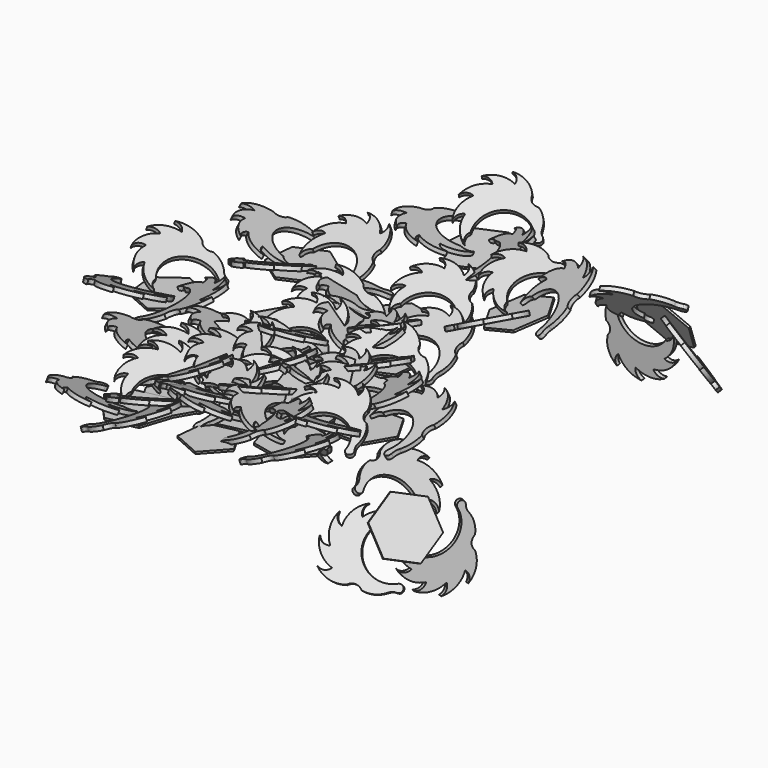
from build123d import *

# Parameters (mm, degrees)
F2_DEPTH  = 1
F3_DEPTH  = 1
F5_COUNT  = 5
F5_ANGLE  = 288
F8_DEPTH  = 2
F9_R      = 5
F11_ANGLE = 65
F12_COUNT = 5
F12_ANGLE = 288
F14_COUNT = 3
F14_ANGLE = 240
F15_COUNT = 5
F15_ANGLE = 288
F16_COUNT = 2
F16_ANGLE = 120
F17_COUNT = 3
F17_ANGLE = 240
F21_COUNT = 3
F21_ANGLE = 144
F25_COUNT = 3
F25_ANGLE = 144
F28_COUNT = 2
F28_ANGLE = 120
F31_COUNT = 3
F31_ANGLE = 144
F35_COUNT = 3
F35_ANGLE = 240
F39_COUNT = 3
F39_ANGLE = 144
F43_COUNT = 3
F43_ANGLE = 144
F47_COUNT = 2
F47_ANGLE = 120
F51_COUNT = 2
F51_ANGLE = 120
F55_COUNT = 2
F55_ANGLE = 120
F59_COUNT = 2
F59_ANGLE = 120


with BuildPart() as f2:
    # F0 (on Top) → F2 (new body)
    with BuildSketch(Plane.XY):
        Polygon((0, -10.3228644035), (7.5, -10.3228644035), (12.1352549156, 3.9429833409), (0, 12.7597621253), align=None)
        Polygon((-7.5, -10.3228644035), (0, -10.3228644035), (0, 12.7597621253), (-12.1352549156, 3.9429833409), align=None)
    extrude(amount=-F2_DEPTH)


with BuildPart() as f3:
    # F1 (on Top) → F3 (new body)
    with BuildSketch(Plane.XY):
        Polygon((32.2091731064, -18.3513614234), (36.844428022, -4.085513679), (26.8074689266, 7.0616587032), (12.1352549156, 3.9429833409), (7.5, -10.3228644035), (17.5369590954, -21.4700367857), align=None)
    extrude(amount=-F3_DEPTH)


with BuildPart() as f5_1:
    # F5: instance of F3
    add(f3.part.rotate(Axis((0, 0, 3.8664315362), (0, 0, 1)), 1 * F5_ANGLE / (F5_COUNT - 1)))


with BuildPart() as f5_2:
    # F5: instance of F3
    add(f3.part.rotate(Axis((0, 0, 3.8664315362), (0, 0, 1)), 2 * F5_ANGLE / (F5_COUNT - 1)))


with BuildPart() as f5_3:
    # F5: instance of F3
    add(f3.part.rotate(Axis((0, 0, 3.8664315362), (0, 0, 1)), 3 * F5_ANGLE / (F5_COUNT - 1)))


with BuildPart() as f5_4:
    # F5: instance of F3
    add(f3.part.rotate(Axis((0, 0, 3.8664315362), (0, 0, 1)), 4 * F5_ANGLE / (F5_COUNT - 1)))


with BuildPart() as f8:
    # F7 (on Right) → F8 (new body)
    with BuildSketch(Plane.YZ):
        with BuildLine():
            ThreePointArc((-24.95999832, 7.9226027528), (-9.4652729948, 14.9790762842), (-1.371596125, 0))
            ThreePointArc((-1.371596125, 0), (1.2710572909, -2.1110060804), (1.0658705895, 1.265065922))
            ThreePointArc((1.0658705895, 1.265065922), (3.462744203, 7.3677169674), (2.5001799222, 13.8531485572))
            ThreePointArc((2.5001799222, 13.8531485572), (0.2653261107, 16.5218708667), (0.7903517664, 19.9629460452))
            ThreePointArc((0.7903517664, 19.9629460452), (-0.5397085451, 26.9271758786), (-5.3926714222, 32.0961514944))
            ThreePointArc((-5.3926714222, 32.0961514944), (-4.1335314331, 29.2501097622), (-5.1634487101, 26.3133330502))
            ThreePointArc((-5.1634487101, 26.3133330502), (-10.3329616952, 31.1657235024), (-17.2973387723, 32.49501261))
            ThreePointArc((-17.2973387723, 32.49501261), (-14.6058117652, 30.9326203981), (-13.7128383045, 27.9513479429))
            ThreePointArc((-13.7128383045, 27.9513479429), (-20.7472257083, 28.8384507879), (-27.1628616524, 25.8203101291))
            ThreePointArc((-27.1628616524, 25.8203101291), (-24.0670194624, 26.1383481587), (-21.5922407749, 24.2513247085))
            ThreePointArc((-21.5922407749, 24.2513247085), (-27.8046056991, 20.834296811), (-31.220945639, 14.6215535346))
            ThreePointArc((-31.220945639, 14.6215535346), (-28.9032947589, 16.6985420881), (-25.7919921886, 16.6265464632))
            ThreePointArc((-25.7919921886, 16.6265464632), (-28.8094223827, 10.2105763396), (-27.9215405786, 3.1762872138))
            ThreePointArc((-27.9215405786, 3.1762872138), (-27.3380736099, 6.1093327886), (-24.95999832, 7.9226027528))
        make_face()
    extrude(amount=-F8_DEPTH)

    # F9
    f9_edges = [f8.edges().sort_by_distance(p)[0] for p in [
        (-1, 1.065871, 1.265066),
    ]]
    fillet(f9_edges, radius=F9_R)


with BuildPart() as f8_1:
    # F11: moved
    add(f8.part.rotate(Axis((0, -11.6566227302, 0), (0, -1, 0)), F11_ANGLE))


with BuildPart() as f12_1:
    # F12: instance of F8
    add(f8_1.part.rotate(Axis((0, 0, 14.2103461549), (0, 0, 1)), 1 * F12_ANGLE / (F12_COUNT - 1)))


with BuildPart() as f12_2:
    # F12: instance of F8
    add(f8_1.part.rotate(Axis((0, 0, 14.2103461549), (0, 0, 1)), 2 * F12_ANGLE / (F12_COUNT - 1)))


with BuildPart() as f12_3:
    # F12: instance of F8
    add(f8_1.part.rotate(Axis((0, 0, 14.2103461549), (0, 0, 1)), 3 * F12_ANGLE / (F12_COUNT - 1)))


with BuildPart() as f12_4:
    # F12: instance of F8
    add(f8_1.part.rotate(Axis((0, 0, 14.2103461549), (0, 0, 1)), 4 * F12_ANGLE / (F12_COUNT - 1)))


with BuildPart() as f14_1:
    # F14: instance of F8
    add(f8_1.part.rotate(Axis((0, -23.3132454603, 7.7419117889), (0, 0, 1)), 1 * F14_ANGLE / (F14_COUNT - 1)))


with BuildPart() as f14_2:
    # F14: instance of F8
    add(f8_1.part.rotate(Axis((0, -23.3132454603, 7.7419117889), (0, 0, 1)), 2 * F14_ANGLE / (F14_COUNT - 1)))


with BuildPart() as f15_1:
    # F15: instance of F14_2
    add(f14_2.part.rotate(Axis((0, 0, 14.2103461549), (0, 0, 1)), 1 * F15_ANGLE / (F15_COUNT - 1)))


with BuildPart() as f15_2:
    # F15: instance of F14_2
    add(f14_2.part.rotate(Axis((0, 0, 14.2103461549), (0, 0, 1)), 2 * F15_ANGLE / (F15_COUNT - 1)))


with BuildPart() as f15_3:
    # F15: instance of F14_2
    add(f14_2.part.rotate(Axis((0, 0, 14.2103461549), (0, 0, 1)), 3 * F15_ANGLE / (F15_COUNT - 1)))


with BuildPart() as f15_4:
    # F15: instance of F14_2
    add(f14_2.part.rotate(Axis((0, 0, 14.2103461549), (0, 0, 1)), 4 * F15_ANGLE / (F15_COUNT - 1)))


with BuildPart() as f15_5:
    # F15: instance of F14_1
    add(f14_1.part.rotate(Axis((0, 0, 14.2103461549), (0, 0, 1)), 1 * F15_ANGLE / (F15_COUNT - 1)))


with BuildPart() as f15_6:
    # F15: instance of F14_1
    add(f14_1.part.rotate(Axis((0, 0, 14.2103461549), (0, 0, 1)), 2 * F15_ANGLE / (F15_COUNT - 1)))


with BuildPart() as f15_7:
    # F15: instance of F14_1
    add(f14_1.part.rotate(Axis((0, 0, 14.2103461549), (0, 0, 1)), 3 * F15_ANGLE / (F15_COUNT - 1)))


with BuildPart() as f15_8:
    # F15: instance of F14_1
    add(f14_1.part.rotate(Axis((0, 0, 14.2103461549), (0, 0, 1)), 4 * F15_ANGLE / (F15_COUNT - 1)))


with BuildPart() as f16_1:
    # F16: instance of F3
    add(f3.part.rotate(Axis((0, -23.3132454603, 7.7419117889), (0, 0, -1)), 1 * F16_ANGLE / (F16_COUNT - 1)))


with BuildPart() as f16_2:
    # F16: instance of F15_5
    add(f15_5.part.rotate(Axis((0, -23.3132454603, 7.7419117889), (0, 0, -1)), 1 * F16_ANGLE / (F16_COUNT - 1)))


with BuildPart() as f16_3:
    # F16: instance of F12_1
    add(f12_1.part.rotate(Axis((0, -23.3132454603, 7.7419117889), (0, 0, -1)), 1 * F16_ANGLE / (F16_COUNT - 1)))


with BuildPart() as f16_4:
    # F16: instance of F15_1
    add(f15_1.part.rotate(Axis((0, -23.3132454603, 7.7419117889), (0, 0, -1)), 1 * F16_ANGLE / (F16_COUNT - 1)))


with BuildPart() as f17_1:
    # F17: instance of F2
    add(f2.part.rotate(Axis((0, -23.3132454603, 7.7419117889), (0, 0, 1)), 1 * F17_ANGLE / (F17_COUNT - 1)))


with BuildPart() as f17_2:
    # F17: instance of F2
    add(f2.part.rotate(Axis((0, -23.3132454603, 7.7419117889), (0, 0, 1)), 2 * F17_ANGLE / (F17_COUNT - 1)))


with BuildPart() as f17_3:
    # F17: instance of F12_2
    add(f12_2.part.rotate(Axis((0, -23.3132454603, 7.7419117889), (0, 0, 1)), 1 * F17_ANGLE / (F17_COUNT - 1)))


with BuildPart() as f17_4:
    # F17: instance of F12_2
    add(f12_2.part.rotate(Axis((0, -23.3132454603, 7.7419117889), (0, 0, 1)), 2 * F17_ANGLE / (F17_COUNT - 1)))


with BuildPart() as f17_5:
    # F17: instance of F12_3
    add(f12_3.part.rotate(Axis((0, -23.3132454603, 7.7419117889), (0, 0, 1)), 1 * F17_ANGLE / (F17_COUNT - 1)))


with BuildPart() as f17_6:
    # F17: instance of F12_3
    add(f12_3.part.rotate(Axis((0, -23.3132454603, 7.7419117889), (0, 0, 1)), 2 * F17_ANGLE / (F17_COUNT - 1)))


with BuildPart() as f21_1:
    # F21: instance of F16_1
    add(f16_1.part.rotate(Axis((-17.4362215627, -33.3800526732, 1.1737770455), (0, 0, -1)), 1 * F21_ANGLE / (F21_COUNT - 1)))


with BuildPart() as f21_2:
    # F21: instance of F16_1
    add(f16_1.part.rotate(Axis((-17.4362215627, -33.3800526732, 1.1737770455), (0, 0, -1)), 2 * F21_ANGLE / (F21_COUNT - 1)))


with BuildPart() as f21_3:
    # F21: instance of F16_3
    add(f16_3.part.rotate(Axis((-17.4362215627, -33.3800526732, 1.1737770455), (0, 0, -1)), 1 * F21_ANGLE / (F21_COUNT - 1)))


with BuildPart() as f21_4:
    # F21: instance of F16_3
    add(f16_3.part.rotate(Axis((-17.4362215627, -33.3800526732, 1.1737770455), (0, 0, -1)), 2 * F21_ANGLE / (F21_COUNT - 1)))


with BuildPart() as f21_5:
    # F21: instance of F16_4
    add(f16_4.part.rotate(Axis((-17.4362215627, -33.3800526732, 1.1737770455), (0, 0, -1)), 1 * F21_ANGLE / (F21_COUNT - 1)))


with BuildPart() as f21_6:
    # F21: instance of F16_4
    add(f16_4.part.rotate(Axis((-17.4362215627, -33.3800526732, 1.1737770455), (0, 0, -1)), 2 * F21_ANGLE / (F21_COUNT - 1)))


with BuildPart() as f21_7:
    # F21: instance of F16_2
    add(f16_2.part.rotate(Axis((-17.4362215627, -33.3800526732, 1.1737770455), (0, 0, -1)), 1 * F21_ANGLE / (F21_COUNT - 1)))


with BuildPart() as f21_8:
    # F21: instance of F16_2
    add(f16_2.part.rotate(Axis((-17.4362215627, -33.3800526732, 1.1737770455), (0, 0, -1)), 2 * F21_ANGLE / (F21_COUNT - 1)))


with BuildPart() as f25_1:
    # F25: instance of F3
    add(f3.part.rotate(Axis((17.4362215627, -33.3800526732, 3.6553055273), (0, 0, -1)), 1 * F25_ANGLE / (F25_COUNT - 1)))


with BuildPart() as f25_2:
    # F25: instance of F3
    add(f3.part.rotate(Axis((17.4362215627, -33.3800526732, 3.6553055273), (0, 0, -1)), 2 * F25_ANGLE / (F25_COUNT - 1)))


with BuildPart() as f25_3:
    # F25: instance of F15_1
    add(f15_1.part.rotate(Axis((17.4362215627, -33.3800526732, 3.6553055273), (0, 0, -1)), 1 * F25_ANGLE / (F25_COUNT - 1)))


with BuildPart() as f25_4:
    # F25: instance of F15_1
    add(f15_1.part.rotate(Axis((17.4362215627, -33.3800526732, 3.6553055273), (0, 0, -1)), 2 * F25_ANGLE / (F25_COUNT - 1)))


with BuildPart() as f25_5:
    # F25: instance of F12_1
    add(f12_1.part.rotate(Axis((17.4362215627, -33.3800526732, 3.6553055273), (0, 0, -1)), 1 * F25_ANGLE / (F25_COUNT - 1)))


with BuildPart() as f25_6:
    # F25: instance of F12_1
    add(f12_1.part.rotate(Axis((17.4362215627, -33.3800526732, 3.6553055273), (0, 0, -1)), 2 * F25_ANGLE / (F25_COUNT - 1)))


with BuildPart() as f25_7:
    # F25: instance of F15_5
    add(f15_5.part.rotate(Axis((17.4362215627, -33.3800526732, 3.6553055273), (0, 0, -1)), 1 * F25_ANGLE / (F25_COUNT - 1)))


with BuildPart() as f25_8:
    # F25: instance of F15_5
    add(f15_5.part.rotate(Axis((17.4362215627, -33.3800526732, 3.6553055273), (0, 0, -1)), 2 * F25_ANGLE / (F25_COUNT - 1)))


with BuildPart() as f28_1:
    # F28: instance of F17_2
    add(f17_2.part.rotate(Axis((0, -50.5694742615, 7.2258593382), (0, 0, -1)), 1 * F28_ANGLE / (F28_COUNT - 1)))


with BuildPart() as f31_1:
    # F31: instance of F25_2
    add(f25_2.part.rotate(Axis((0, -75.8542113922, -11.0916886207), (0, 0, 1)), 1 * F31_ANGLE / (F31_COUNT - 1)))


with BuildPart() as f31_2:
    # F31: instance of F25_2
    add(f25_2.part.rotate(Axis((0, -75.8542113922, -11.0916886207), (0, 0, 1)), 2 * F31_ANGLE / (F31_COUNT - 1)))


with BuildPart() as f31_3:
    # F31: instance of F25_4
    add(f25_4.part.rotate(Axis((0, -75.8542113922, -11.0916886207), (0, 0, 1)), 1 * F31_ANGLE / (F31_COUNT - 1)))


with BuildPart() as f31_4:
    # F31: instance of F25_4
    add(f25_4.part.rotate(Axis((0, -75.8542113922, -11.0916886207), (0, 0, 1)), 2 * F31_ANGLE / (F31_COUNT - 1)))


with BuildPart() as f31_5:
    # F31: instance of F25_6
    add(f25_6.part.rotate(Axis((0, -75.8542113922, -11.0916886207), (0, 0, 1)), 1 * F31_ANGLE / (F31_COUNT - 1)))


with BuildPart() as f31_6:
    # F31: instance of F25_6
    add(f25_6.part.rotate(Axis((0, -75.8542113922, -11.0916886207), (0, 0, 1)), 2 * F31_ANGLE / (F31_COUNT - 1)))


with BuildPart() as f31_7:
    # F31: instance of F17_4
    add(f17_4.part.rotate(Axis((0, -75.8542113922, -11.0916886207), (0, 0, 1)), 1 * F31_ANGLE / (F31_COUNT - 1)))


with BuildPart() as f31_8:
    # F31: instance of F17_4
    add(f17_4.part.rotate(Axis((0, -75.8542113922, -11.0916886207), (0, 0, 1)), 2 * F31_ANGLE / (F31_COUNT - 1)))


with BuildPart() as f35_1:
    # F35: instance of F2
    add(f2.part.rotate(Axis((-13.7031818646, 18.8608117714, 14.763216387), (0, 0, -1)), 1 * F35_ANGLE / (F35_COUNT - 1)))


with BuildPart() as f35_2:
    # F35: instance of F2
    add(f2.part.rotate(Axis((-13.7031818646, 18.8608117714, 14.763216387), (0, 0, -1)), 2 * F35_ANGLE / (F35_COUNT - 1)))


with BuildPart() as f39_1:
    # F39: instance of F21_2
    add(f21_2.part.rotate(Axis((-36.888714927, 16.4239140497, 16.806895229), (0, 0, -1)), 1 * F39_ANGLE / (F39_COUNT - 1)))


with BuildPart() as f39_2:
    # F39: instance of F21_2
    add(f21_2.part.rotate(Axis((-36.888714927, 16.4239140497, 16.806895229), (0, 0, -1)), 2 * F39_ANGLE / (F39_COUNT - 1)))


with BuildPart() as f39_3:
    # F39: instance of F21_6
    add(f21_6.part.rotate(Axis((-36.888714927, 16.4239140497, 16.806895229), (0, 0, -1)), 1 * F39_ANGLE / (F39_COUNT - 1)))


with BuildPart() as f39_4:
    # F39: instance of F21_6
    add(f21_6.part.rotate(Axis((-36.888714927, 16.4239140497, 16.806895229), (0, 0, -1)), 2 * F39_ANGLE / (F39_COUNT - 1)))


with BuildPart() as f39_5:
    # F39: instance of F21_4
    add(f21_4.part.rotate(Axis((-36.888714927, 16.4239140497, 16.806895229), (0, 0, -1)), 1 * F39_ANGLE / (F39_COUNT - 1)))


with BuildPart() as f39_6:
    # F39: instance of F21_4
    add(f21_4.part.rotate(Axis((-36.888714927, 16.4239140497, 16.806895229), (0, 0, -1)), 2 * F39_ANGLE / (F39_COUNT - 1)))


with BuildPart() as f39_7:
    # F39: instance of F17_3
    add(f17_3.part.rotate(Axis((-36.888714927, 16.4239140497, 16.806895229), (0, 0, -1)), 1 * F39_ANGLE / (F39_COUNT - 1)))


with BuildPart() as f39_8:
    # F39: instance of F17_3
    add(f17_3.part.rotate(Axis((-36.888714927, 16.4239140497, 16.806895229), (0, 0, -1)), 2 * F39_ANGLE / (F39_COUNT - 1)))


with BuildPart() as f43_1:
    # F43: instance of F39_2
    add(f39_2.part.rotate(Axis((-8.0111221618, 39.3528699367, 26.0918540489), (0.1436912512, 0.0305425183, -0.9891511406)), 1 * F43_ANGLE / (F43_COUNT - 1)))


with BuildPart() as f43_2:
    # F43: instance of F39_2
    add(f39_2.part.rotate(Axis((-8.0111221618, 39.3528699367, 26.0918540489), (0.1436912512, 0.0305425183, -0.9891511406)), 2 * F43_ANGLE / (F43_COUNT - 1)))


with BuildPart() as f43_3:
    # F43: instance of F39_6
    add(f39_6.part.rotate(Axis((-8.0111221618, 39.3528699367, 26.0918540489), (0.1436912512, 0.0305425183, -0.9891511406)), 1 * F43_ANGLE / (F43_COUNT - 1)))


with BuildPart() as f43_4:
    # F43: instance of F39_6
    add(f39_6.part.rotate(Axis((-8.0111221618, 39.3528699367, 26.0918540489), (0.1436912512, 0.0305425183, -0.9891511406)), 2 * F43_ANGLE / (F43_COUNT - 1)))


with BuildPart() as f43_5:
    # F43: instance of F39_8
    add(f39_8.part.rotate(Axis((-8.0111221618, 39.3528699367, 26.0918540489), (0.1436912512, 0.0305425183, -0.9891511406)), 1 * F43_ANGLE / (F43_COUNT - 1)))


with BuildPart() as f43_6:
    # F43: instance of F39_8
    add(f39_8.part.rotate(Axis((-8.0111221618, 39.3528699367, 26.0918540489), (0.1436912512, 0.0305425183, -0.9891511406)), 2 * F43_ANGLE / (F43_COUNT - 1)))


with BuildPart() as f43_7:
    # F43: instance of F39_4
    add(f39_4.part.rotate(Axis((-8.0111221618, 39.3528699367, 26.0918540489), (0.1436912512, 0.0305425183, -0.9891511406)), 1 * F43_ANGLE / (F43_COUNT - 1)))


with BuildPart() as f43_8:
    # F43: instance of F39_4
    add(f39_4.part.rotate(Axis((-8.0111221618, 39.3528699367, 26.0918540489), (0.1436912512, 0.0305425183, -0.9891511406)), 2 * F43_ANGLE / (F43_COUNT - 1)))


with BuildPart() as f47_1:
    # F47: instance of F21_2
    add(f21_2.part.rotate(Axis((-92.9675551418, 6.3909135689, 0), (0.9981475566, 0.0608395868, 0)), 1 * F47_ANGLE / (F47_COUNT - 1)))


with BuildPart() as f47_2:
    # F47: instance of F21_4
    add(f21_4.part.rotate(Axis((-92.9675551418, 6.3909135689, 0), (0.9981475566, 0.0608395868, 0)), 1 * F47_ANGLE / (F47_COUNT - 1)))


with BuildPart() as f47_3:
    # F47: instance of F21_6
    add(f21_6.part.rotate(Axis((-92.9675551418, 6.3909135689, 0), (0.9981475566, 0.0608395868, 0)), 1 * F47_ANGLE / (F47_COUNT - 1)))


with BuildPart() as f47_4:
    # F47: instance of F17_3
    add(f17_3.part.rotate(Axis((-92.9675551418, 6.3909135689, 0), (0.9981475566, 0.0608395868, 0)), 1 * F47_ANGLE / (F47_COUNT - 1)))


with BuildPart() as f51_1:
    # F51: instance of F15_5
    add(f15_5.part.rotate(Axis((54.8325005267, -26.1451923699, 0), (-0.5517624006, -0.8340013509, 0)), 1 * F51_ANGLE / (F51_COUNT - 1)))


with BuildPart() as f51_2:
    # F51: instance of F12_1
    add(f12_1.part.rotate(Axis((54.8325005267, -26.1451923699, 0), (-0.5517624006, -0.8340013509, 0)), 1 * F51_ANGLE / (F51_COUNT - 1)))


with BuildPart() as f51_3:
    # F51: instance of F15_1
    add(f15_1.part.rotate(Axis((54.8325005267, -26.1451923699, 0), (-0.5517624006, -0.8340013509, 0)), 1 * F51_ANGLE / (F51_COUNT - 1)))


with BuildPart() as f51_4:
    # F51: instance of F3
    add(f3.part.rotate(Axis((54.8325005267, -26.1451923699, 0), (-0.5517624006, -0.8340013509, 0)), 1 * F51_ANGLE / (F51_COUNT - 1)))


with BuildPart() as f55_1:
    # F55: instance of F25_2
    add(f25_2.part.rotate(Axis((-16.1490089096, -14.5711711071, -22.7108248674), (0, 0, 1)), 1 * F55_ANGLE / (F55_COUNT - 1)))


with BuildPart() as f55_2:
    # F55: instance of F25_4
    add(f25_4.part.rotate(Axis((-16.1490089096, -14.5711711071, -22.7108248674), (0, 0, 1)), 1 * F55_ANGLE / (F55_COUNT - 1)))


with BuildPart() as f55_3:
    # F55: instance of F25_6
    add(f25_6.part.rotate(Axis((-16.1490089096, -14.5711711071, -22.7108248674), (0, 0, 1)), 1 * F55_ANGLE / (F55_COUNT - 1)))


with BuildPart() as f55_4:
    # F55: instance of F17_4
    add(f17_4.part.rotate(Axis((-16.1490089096, -14.5711711071, -22.7108248674), (0, 0, 1)), 1 * F55_ANGLE / (F55_COUNT - 1)))


with BuildPart() as f59_1:
    # F59: instance of F51_4
    add(f51_4.part.rotate(Axis((-1.4890504043, 51.0498282433, -7.9085918438), (0, 0, 1)), 1 * F59_ANGLE / (F59_COUNT - 1)))


with BuildPart() as f59_2:
    # F59: instance of F51_3
    add(f51_3.part.rotate(Axis((-1.4890504043, 51.0498282433, -7.9085918438), (0, 0, 1)), 1 * F59_ANGLE / (F59_COUNT - 1)))


with BuildPart() as f59_3:
    # F59: instance of F51_1
    add(f51_1.part.rotate(Axis((-1.4890504043, 51.0498282433, -7.9085918438), (0, 0, 1)), 1 * F59_ANGLE / (F59_COUNT - 1)))


with BuildPart() as f59_4:
    # F59: instance of F51_2
    add(f51_2.part.rotate(Axis((-1.4890504043, 51.0498282433, -7.9085918438), (0, 0, 1)), 1 * F59_ANGLE / (F59_COUNT - 1)))


solid = Compound([f2.part, f3.part, f5_1.part, f5_2.part, f5_3.part, f5_4.part, f8_1.part, f12_1.part, f12_2.part, f12_3.part, f12_4.part, f14_1.part, f14_2.part, f15_1.part, f15_2.part, f15_3.part, f15_4.part, f15_5.part, f15_6.part, f15_7.part, f15_8.part, f16_1.part, f16_2.part, f16_3.part, f16_4.part, f17_1.part, f17_2.part, f17_3.part, f17_4.part, f17_5.part, f17_6.part, f21_1.part, f21_2.part, f21_3.part, f21_4.part, f21_5.part, f21_6.part, f25_1.part, f25_2.part, f25_3.part, f25_4.part, f25_5.part, f25_6.part, f28_1.part, f31_1.part, f31_2.part, f31_3.part, f31_4.part, f31_5.part, f31_6.part, f31_7.part, f31_8.part, f35_1.part, f35_2.part, f39_1.part, f39_2.part, f39_3.part, f39_4.part, f39_5.part, f39_6.part, f39_7.part, f39_8.part, f43_1.part, f43_2.part, f43_3.part, f43_4.part, f43_5.part, f43_6.part, f43_7.part, f43_8.part, f47_1.part, f47_2.part, f47_3.part, f47_4.part, f51_1.part, f51_2.part, f51_3.part, f51_4.part, f55_1.part, f55_2.part, f55_3.part, f55_4.part, f59_1.part, f59_2.part, f59_3.part, f59_4.part])
